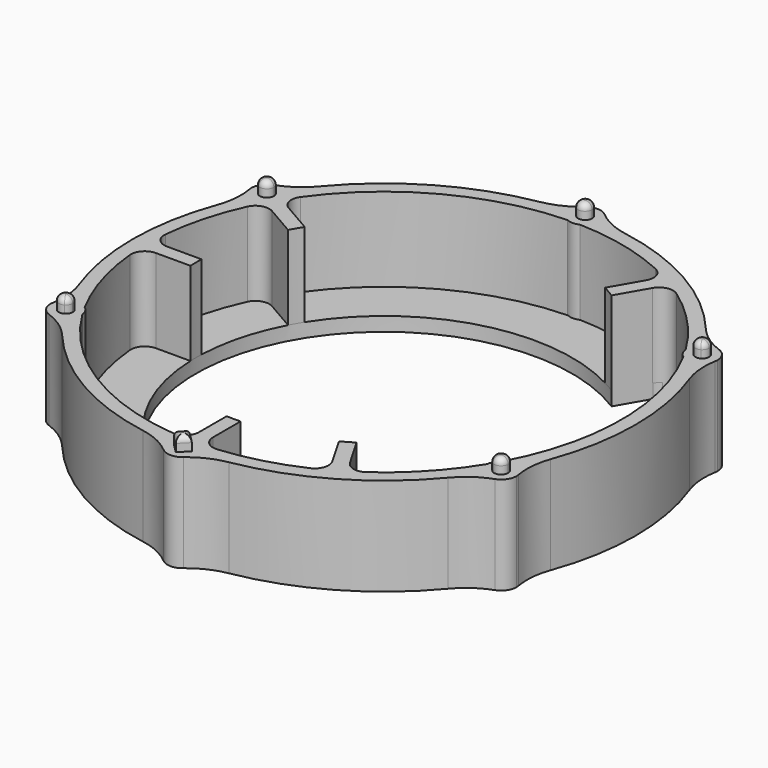
from build123d import *

# Parameters (mm, degrees)
F1_R          = 18
F1_R_2        = 17
F2_DEPTH      = 7
F3_DEPTH      = 7
F4_DEPTH      = 1
F6_DEPTH      = 7
F7_R          = 1
F8_R          = 5
F9_DEPTH      = 8
F10_R         = 0.44999
F11_DEPTH     = 1.8
F13_DEPTH     = 1
F12_R         = 13.47
F14_DEPTH     = 1
F15_T1_DEPTH  = 1
F15_T6_DEPTH  = 3.7422914514
F15_S7_R      = 1
F15_T8_DEPTH  = 4
F15_T12_DEPTH = 3.7422914514
F15_S13_R     = 1
F15_T14_DEPTH = 4
F15_T18_DEPTH = 3.7422914514
F15_S19_R     = 1
F15_T20_DEPTH = 4


# Not quite as in the source:
# - a fillet or chamfer that OpenCascade refuses, or shapes differently, is made with other operations: its cross-section is extruded or revolved along the edge and cut away or added
# - a fillet or chamfer is up to 0.001 mm smaller than in the source, because OpenCascade refuses the exact size


with BuildPart() as f2:
    # F1 (on Top) → F2 (new body)
    with BuildSketch(Plane.XY):
        Circle(F1_R)
        Circle(F1_R_2, mode=Mode.SUBTRACT)
    extrude(amount=F2_DEPTH)

    # F0 (on Top) → F3 (join)
    with BuildSketch(Plane.XY):
        with BuildLine():
            Line((-11.4073228059, 7.1633711619), (-14.4660626528, 8.9293354359))
            ThreePointArc((-14.4660626528, 8.9293354359), (-14.7224318643, 8.5), (-14.9660626528, 8.0633100321))
            Line((-14.9660626528, 8.0633100321), (-11.9073228059, 6.2973457581))
            ThreePointArc((-11.9073228059, 6.2973457581), (-11.665362189, 6.735), (-11.4073228059, 7.1633711619))
        make_face()
        with BuildLine():
            Line((7.1633711619, 11.4073228059), (8.9293354359, 14.4660626528))
            ThreePointArc((8.9293354359, 14.4660626528), (8.5, 14.7224318643), (8.0633100321, 14.9660626528))
            Line((8.0633100321, 14.9660626528), (6.2973457581, 11.9073228059))
            ThreePointArc((6.2973457581, 11.9073228059), (6.735, 11.665362189), (7.1633711619, 11.4073228059))
        make_face()
        with BuildLine():
            ThreePointArc((-0.5, -16.992645468), (0, -17), (0.5, -16.992645468))
            Line((0.5, -16.992645468), (0.5, -13.46071692))
            ThreePointArc((0.5, -13.46071692), (0, -13.47), (-0.5, -13.46071692))
            Line((-0.5, -13.46071692), (-0.5, -16.992645468))
        make_face()
        with BuildLine():
            ThreePointArc((8.0633100321, -14.9660626528), (8.5, -14.7224318643), (8.9293354359, -14.4660626528))
            Line((8.9293354359, -14.4660626528), (7.1633711619, -11.4073228059))
            ThreePointArc((7.1633711619, -11.4073228059), (6.735, -11.665362189), (6.2973457581, -11.9073228059))
            Line((6.2973457581, -11.9073228059), (8.0633100321, -14.9660626528))
        make_face()
        with BuildLine():
            Line((-13.46071692, 0.5), (-16.992645468, 0.5))
            ThreePointArc((-16.992645468, 0.5), (-17, 0), (-16.992645468, -0.5))
            Line((-16.992645468, -0.5), (-13.46071692, -0.5))
            ThreePointArc((-13.46071692, -0.5), (-13.47, 0), (-13.46071692, 0.5))
        make_face()
    extrude(amount=F3_DEPTH)

    # F1 (on Top) → F4 (join)
    with BuildSketch(Plane.XY):
        Circle(F1_R)
        Circle(F1_R_2, mode=Mode.SUBTRACT)
        Circle(F1_R_2)
    extrude(amount=F4_DEPTH)

    # F5 (on Top) → F6 (join)
    with BuildSketch(Plane.XY):
        with BuildLine():
            ThreePointArc((-14.4884572681, 9), (-14.6275367743, 9.5353800561), (-15.0096060035, 9.935377578))
            ThreePointArc((-15.0096060035, 9.935377578), (-15.1731450826, 9.6837837802), (-15.3324673166, 9.4294987133))
            ThreePointArc((-15.3324673166, 9.4294987133), (-15.153718855, 9.2469868663), (-15.0884572681, 9))
            ThreePointArc((-15.0884572681, 9), (-15.3354561915, 8.5687338928), (-15.832419089, 8.5635568422))
            ThreePointArc((-15.832419089, 8.5635568422), (-15.9729752997, 8.2984372068), (-16.1090923805, 8.0310113108))
            ThreePointArc((-16.1090923805, 8.0310113108), (-15.0239657375, 8.0558870238), (-14.4884572681, 9))
        make_face()
        with BuildLine():
            ThreePointArc((-15.3324673166, 9.4294987133), (-15.1731450826, 9.6837837802), (-15.0096060035, 9.935377578))
            ThreePointArc((-15.0096060035, 9.935377578), (-16.5410852123, 9.55), (-16.1090923805, 8.0310113108))
            ThreePointArc((-16.1090923805, 8.0310113108), (-15.9729752997, 8.2984372068), (-15.832419089, 8.5635568422))
            ThreePointArc((-15.832419089, 8.5635568422), (-16.02146997, 9.25), (-15.3324673166, 9.4294987133))
        make_face()
        with BuildLine():
            ThreePointArc((-1.099486377, 17.9663888889), (0, 16.9), (1.099486377, 17.9663888889))
            ThreePointArc((1.099486377, 17.9663888889), (0.7998302171, 17.982220987), (0.4999517724, 17.9930555556))
            ThreePointArc((0.4999517724, 17.9930555556), (0, 17.5), (-0.4999517724, 17.9930555556))
            ThreePointArc((-0.4999517724, 17.9930555556), (-0.7998302171, 17.982220987), (-1.099486377, 17.9663888889))
        make_face()
        with BuildLine():
            ThreePointArc((0.4999517724, 17.9930555556), (0.7998302171, 17.982220987), (1.099486377, 17.9663888889))
            ThreePointArc((1.099486377, 17.9663888889), (1.0998715868, 17.9831924823), (1.1, 18))
            ThreePointArc((1.1, 18), (-0.0168075177, 19.0998715868), (-1.099486377, 17.9663888889))
            ThreePointArc((-1.099486377, 17.9663888889), (-0.7998302171, 17.982220987), (-0.4999517724, 17.9930555556))
            ThreePointArc((-0.4999517724, 17.9930555556), (-0.003472306, 18.4999879429), (0.5, 18))
            ThreePointArc((0.5, 18), (0.4999879429, 17.996527694), (0.4999517724, 17.9930555556))
        make_face()
        with BuildLine():
            ThreePointArc((15.832419089, 8.5635568422), (15.9729752997, 8.2984372068), (16.1090923805, 8.0310113108))
            ThreePointArc((16.1090923805, 8.0310113108), (16.5325702443, 8.4355084694), (16.6884572681, 9))
            ThreePointArc((16.6884572681, 9), (16.1238373242, 9.9609204939), (15.0096060035, 9.935377578))
            ThreePointArc((15.0096060035, 9.935377578), (15.1731450826, 9.6837837802), (15.3324673166, 9.4294987133))
            ThreePointArc((15.3324673166, 9.4294987133), (15.8354441344, 9.4347384132), (16.0884572681, 9))
            ThreePointArc((16.0884572681, 9), (16.0197233753, 8.7469989234), (15.832419089, 8.5635568422))
        make_face()
        with BuildLine():
            ThreePointArc((15.0096060035, 9.935377578), (14.635829324, 8.45), (16.1090923805, 8.0310113108))
            ThreePointArc((16.1090923805, 8.0310113108), (15.9729752997, 8.2984372068), (15.832419089, 8.5635568422))
            ThreePointArc((15.832419089, 8.5635568422), (15.1554445662, 8.75), (15.3324673166, 9.4294987133))
            ThreePointArc((15.3324673166, 9.4294987133), (15.1731450826, 9.6837837802), (15.0096060035, 9.935377578))
        make_face()
        with BuildLine():
            ThreePointArc((-15.3324673166, -9.4294987133), (-15.1731450826, -9.6837837802), (-15.0096060035, -9.935377578))
            ThreePointArc((-15.0096060035, -9.935377578), (-14.6275367743, -9.5353800561), (-14.4884572681, -9))
            ThreePointArc((-14.4884572681, -9), (-15.0239657375, -8.0558870238), (-16.1090923805, -8.0310113108))
            ThreePointArc((-16.1090923805, -8.0310113108), (-15.9729752997, -8.2984372068), (-15.832419089, -8.5635568422))
            ThreePointArc((-15.832419089, -8.5635568422), (-15.3354561915, -8.5687338928), (-15.0884572681, -9))
            ThreePointArc((-15.0884572681, -9), (-15.153718855, -9.2469868663), (-15.3324673166, -9.4294987133))
        make_face()
        with BuildLine():
            ThreePointArc((-16.1090923805, -8.0310113108), (-16.5410852123, -9.55), (-15.0096060035, -9.935377578))
            ThreePointArc((-15.0096060035, -9.935377578), (-15.1731450826, -9.6837837802), (-15.3324673166, -9.4294987133))
            ThreePointArc((-15.3324673166, -9.4294987133), (-16.02146997, -9.25), (-15.832419089, -8.5635568422))
            ThreePointArc((-15.832419089, -8.5635568422), (-15.9729752997, -8.2984372068), (-16.1090923805, -8.0310113108))
        make_face()
        with BuildLine():
            ThreePointArc((0.6255239257, -17.9891278226), (0.8625800837, -17.9793202207), (1.099486377, -17.9663888889))
            ThreePointArc((1.099486377, -17.9663888889), (0, -16.9), (-1.099486377, -17.9663888889))
            ThreePointArc((-1.099486377, -17.9663888889), (-0.8625800837, -17.9793202207), (-0.6255239257, -17.9891278226))
            Line((-0.6255239257, -17.9891278226), (0, -17.3636038969))
            Line((0, -17.3636038969), (0.6255239257, -17.9891278226))
        make_face()
        with BuildLine():
            ThreePointArc((1.1, -18), (1.0998715868, -17.9831924823), (1.099486377, -17.9663888889))
            ThreePointArc((1.099486377, -17.9663888889), (0.8625800837, -17.9793202207), (0.6255239257, -17.9891278226))
            Line((0.6255239257, -17.9891278226), (0.6363961031, -18))
            Line((0.6363961031, -18), (0, -18.6363961031))
            Line((0, -18.6363961031), (-0.6363961031, -18))
            Line((-0.6363961031, -18), (-0.6255239257, -17.9891278226))
            ThreePointArc((-0.6255239257, -17.9891278226), (-0.8625800837, -17.9793202207), (-1.099486377, -17.9663888889))
            ThreePointArc((-1.099486377, -17.9663888889), (-0.0168075177, -19.0998715868), (1.1, -18))
        make_face()
        with BuildLine():
            ThreePointArc((16.6884572681, -9), (16.5325702443, -8.4355084694), (16.1090923805, -8.0310113108))
            ThreePointArc((16.1090923805, -8.0310113108), (15.9729752997, -8.2984372068), (15.832419089, -8.5635568422))
            ThreePointArc((15.832419089, -8.5635568422), (16.0197233753, -8.7469989234), (16.0884572681, -9))
            ThreePointArc((16.0884572681, -9), (15.8354441344, -9.4347384132), (15.3324673166, -9.4294987133))
            ThreePointArc((15.3324673166, -9.4294987133), (15.1731450826, -9.6837837802), (15.0096060035, -9.935377578))
            ThreePointArc((15.0096060035, -9.935377578), (16.1238373242, -9.9609204939), (16.6884572681, -9))
        make_face()
        with BuildLine():
            ThreePointArc((15.832419089, -8.5635568422), (15.9729752997, -8.2984372068), (16.1090923805, -8.0310113108))
            ThreePointArc((16.1090923805, -8.0310113108), (14.635829324, -8.45), (15.0096060035, -9.935377578))
            ThreePointArc((15.0096060035, -9.935377578), (15.1731450826, -9.6837837802), (15.3324673166, -9.4294987133))
            ThreePointArc((15.3324673166, -9.4294987133), (15.1554445662, -8.75), (15.832419089, -8.5635568422))
        make_face()
        with BuildLine():
            ThreePointArc((-15.0884572681, 9), (-15.153718855, 9.2469868663), (-15.3324673166, 9.4294987133))
            ThreePointArc((-15.3324673166, 9.4294987133), (-15.5884572681, 9), (-15.832419089, 8.5635568422))
            ThreePointArc((-15.832419089, 8.5635568422), (-15.3354561915, 8.5687338928), (-15.0884572681, 9))
        make_face()
        with BuildLine():
            ThreePointArc((-15.832419089, 8.5635568422), (-15.5884572681, 9), (-15.3324673166, 9.4294987133))
            ThreePointArc((-15.3324673166, 9.4294987133), (-16.02146997, 9.25), (-15.832419089, 8.5635568422))
        make_face()
        with BuildLine():
            ThreePointArc((-0.4999517724, 17.9930555556), (0, 18), (0.4999517724, 17.9930555556))
            ThreePointArc((0.4999517724, 17.9930555556), (0.4999879429, 17.996527694), (0.5, 18))
            ThreePointArc((0.5, 18), (-0.003472306, 18.4999879429), (-0.4999517724, 17.9930555556))
        make_face()
        with BuildLine():
            ThreePointArc((-0.4999517724, 17.9930555556), (0, 17.5), (0.4999517724, 17.9930555556))
            ThreePointArc((0.4999517724, 17.9930555556), (0, 18), (-0.4999517724, 17.9930555556))
        make_face()
        with BuildLine():
            ThreePointArc((15.3324673166, 9.4294987133), (15.5884572681, 9), (15.832419089, 8.5635568422))
            ThreePointArc((15.832419089, 8.5635568422), (16.0197233753, 8.7469989234), (16.0884572681, 9))
            ThreePointArc((16.0884572681, 9), (15.8354441344, 9.4347384132), (15.3324673166, 9.4294987133))
        make_face()
        with BuildLine():
            ThreePointArc((15.3324673166, 9.4294987133), (15.1554445662, 8.75), (15.832419089, 8.5635568422))
            ThreePointArc((15.832419089, 8.5635568422), (15.5884572681, 9), (15.3324673166, 9.4294987133))
        make_face()
        with BuildLine():
            ThreePointArc((16.0884572681, -9), (16.0197233753, -8.7469989234), (15.832419089, -8.5635568422))
            ThreePointArc((15.832419089, -8.5635568422), (15.5884572681, -9), (15.3324673166, -9.4294987133))
            ThreePointArc((15.3324673166, -9.4294987133), (15.8354441344, -9.4347384132), (16.0884572681, -9))
        make_face()
        with BuildLine():
            ThreePointArc((15.3324673166, -9.4294987133), (15.5884572681, -9), (15.832419089, -8.5635568422))
            ThreePointArc((15.832419089, -8.5635568422), (15.1554445662, -8.75), (15.3324673166, -9.4294987133))
        make_face()
        with BuildLine():
            Line((0.6363961031, -18), (0.6255239257, -17.9891278226))
            ThreePointArc((0.6255239257, -17.9891278226), (0, -18), (-0.6255239257, -17.9891278226))
            Line((-0.6255239257, -17.9891278226), (-0.6363961031, -18))
            Line((-0.6363961031, -18), (0, -18.6363961031))
            Line((0, -18.6363961031), (0.6363961031, -18))
        make_face()
        with BuildLine():
            ThreePointArc((-15.832419089, -8.5635568422), (-16.02146997, -9.25), (-15.3324673166, -9.4294987133))
            ThreePointArc((-15.3324673166, -9.4294987133), (-15.5884572681, -9), (-15.832419089, -8.5635568422))
        make_face()
        with BuildLine():
            ThreePointArc((-15.832419089, -8.5635568422), (-15.5884572681, -9), (-15.3324673166, -9.4294987133))
            ThreePointArc((-15.3324673166, -9.4294987133), (-15.153718855, -9.2469868663), (-15.0884572681, -9))
            ThreePointArc((-15.0884572681, -9), (-15.3354561915, -8.5687338928), (-15.832419089, -8.5635568422))
        make_face()
        with BuildLine():
            ThreePointArc((-0.6255239257, -17.9891278226), (0, -18), (0.6255239257, -17.9891278226))
            Line((0.6255239257, -17.9891278226), (0, -17.3636038969))
            Line((0, -17.3636038969), (-0.6255239257, -17.9891278226))
        make_face()
    extrude(amount=F6_DEPTH)

    # F7
    f7_edges = [f2.edges().sort_by_distance(p)[0] for p in [
        (0.5, -16.992645, 4),
        (8.06331, 14.966063, 4),
        (-16.992645, 0.5, 4),
        (8.929335, -14.466063, 4),
        (-14.466063, 8.929335, 4),
        (-0.5, -16.992645, 4),
        (-16.992645, -0.5, 4),
        (-14.966063, 8.06331, 4),
        (8.06331, -14.966063, 4),
        (8.929335, 14.466063, 4),
    ]]
    fillet(f7_edges, radius=F7_R)

    # F8 (call 1 of 12: OpenCascade refuses the feature's edges together)
    f8_edges = [f2.edges().sort_by_distance(p)[0] for p in [
        (-16.109092, 8.031011, 3.5),
    ]]
    fillet(f8_edges, radius=F8_R)

    # F8#2 (call 2 of 12)
    f8_2_edges = [f2.edges().sort_by_distance(p)[0] for p in [
        (-15.009606, 9.935378, 3.5),
    ]]
    fillet(f8_2_edges, radius=F8_R)

    # F8#3 (call 3 of 12)
    f8_3_edges = [f2.edges().sort_by_distance(p)[0] for p in [
        (-1.099486, 17.966389, 3.5),
    ]]
    fillet(f8_3_edges, radius=F8_R)

    # F8#4 (call 4 of 12)
    f8_4_edges = [f2.edges().sort_by_distance(p)[0] for p in [
        (1.099486, 17.966389, 3.5),
    ]]
    fillet(f8_4_edges, radius=F8_R)

    # F8#5 (call 5 of 12)
    f8_5_edges = [f2.edges().sort_by_distance(p)[0] for p in [
        (-15.009606, -9.935378, 3.5),
    ]]
    fillet(f8_5_edges, radius=F8_R)

    # F8#6 (call 6 of 12)
    f8_6_edges = [f2.edges().sort_by_distance(p)[0] for p in [
        (-16.109092, -8.031011, 3.5),
    ]]
    fillet(f8_6_edges, radius=F8_R)

    # F8#7 (call 7 of 12)
    f8_7_edges = [f2.edges().sort_by_distance(p)[0] for p in [
        (1.099486, -17.966389, 3.5),
    ]]
    fillet(f8_7_edges, radius=F8_R)

    # F8#8 (call 8 of 12)
    f8_8_edges = [f2.edges().sort_by_distance(p)[0] for p in [
        (-1.099486, -17.966389, 3.5),
    ]]
    fillet(f8_8_edges, radius=F8_R)

    # F8#10 (call 9 of 12)
    f8_10_edges = [f2.edges().sort_by_distance(p)[0] for p in [
        (15.009606, -9.935378, 3.5),
    ]]
    fillet(f8_10_edges, radius=F8_R)

    # F8#11 (call 10 of 12)
    f8_11_edges = [f2.edges().sort_by_distance(p)[0] for p in [
        (16.109092, 8.031011, 3.5),
    ]]
    fillet(f8_11_edges, radius=F8_R)

    # F8#12 (call 11 of 12)
    f8_12_edges = [f2.edges().sort_by_distance(p)[0] for p in [
        (15.009606, 9.935378, 3.5),
    ]]
    fillet(f8_12_edges, radius=F8_R)

    # F8#9 (call 12 of 12)
    f8_9_edges = [f2.edges().sort_by_distance(p)[0] for p in [
        (16.109092, -8.031011, 3.5),
    ]]
    fillet(f8_9_edges, radius=F8_R)

    # F5 (on Top) → F9 (join)
    with BuildSketch(Plane.XY):
        with BuildLine():
            ThreePointArc((-15.832419089, 8.5635568422), (-15.5884572681, 9), (-15.3324673166, 9.4294987133))
            ThreePointArc((-15.3324673166, 9.4294987133), (-16.02146997, 9.25), (-15.832419089, 8.5635568422))
        make_face()
        with BuildLine():
            ThreePointArc((-15.0884572681, 9), (-15.153718855, 9.2469868663), (-15.3324673166, 9.4294987133))
            ThreePointArc((-15.3324673166, 9.4294987133), (-15.5884572681, 9), (-15.832419089, 8.5635568422))
            ThreePointArc((-15.832419089, 8.5635568422), (-15.3354561915, 8.5687338928), (-15.0884572681, 9))
        make_face()
        with BuildLine():
            ThreePointArc((-0.4999517724, 17.9930555556), (0, 18), (0.4999517724, 17.9930555556))
            ThreePointArc((0.4999517724, 17.9930555556), (0.4999879429, 17.996527694), (0.5, 18))
            ThreePointArc((0.5, 18), (-0.003472306, 18.4999879429), (-0.4999517724, 17.9930555556))
        make_face()
        with BuildLine():
            ThreePointArc((-0.4999517724, 17.9930555556), (0, 17.5), (0.4999517724, 17.9930555556))
            ThreePointArc((0.4999517724, 17.9930555556), (0, 18), (-0.4999517724, 17.9930555556))
        make_face()
        with BuildLine():
            ThreePointArc((15.3324673166, 9.4294987133), (15.1554445662, 8.75), (15.832419089, 8.5635568422))
            ThreePointArc((15.832419089, 8.5635568422), (15.5884572681, 9), (15.3324673166, 9.4294987133))
        make_face()
        with BuildLine():
            ThreePointArc((15.3324673166, 9.4294987133), (15.5884572681, 9), (15.832419089, 8.5635568422))
            ThreePointArc((15.832419089, 8.5635568422), (16.0197233753, 8.7469989234), (16.0884572681, 9))
            ThreePointArc((16.0884572681, 9), (15.8354441344, 9.4347384132), (15.3324673166, 9.4294987133))
        make_face()
        with BuildLine():
            ThreePointArc((15.3324673166, -9.4294987133), (15.5884572681, -9), (15.832419089, -8.5635568422))
            ThreePointArc((15.832419089, -8.5635568422), (15.1554445662, -8.75), (15.3324673166, -9.4294987133))
        make_face()
        with BuildLine():
            ThreePointArc((16.0884572681, -9), (16.0197233753, -8.7469989234), (15.832419089, -8.5635568422))
            ThreePointArc((15.832419089, -8.5635568422), (15.5884572681, -9), (15.3324673166, -9.4294987133))
            ThreePointArc((15.3324673166, -9.4294987133), (15.8354441344, -9.4347384132), (16.0884572681, -9))
        make_face()
        with BuildLine():
            Line((0.6363961031, -18), (0.6255239257, -17.9891278226))
            ThreePointArc((0.6255239257, -17.9891278226), (0, -18), (-0.6255239257, -17.9891278226))
            Line((-0.6255239257, -17.9891278226), (-0.6363961031, -18))
            Line((-0.6363961031, -18), (0, -18.6363961031))
            Line((0, -18.6363961031), (0.6363961031, -18))
        make_face()
        with BuildLine():
            ThreePointArc((-0.6255239257, -17.9891278226), (0, -18), (0.6255239257, -17.9891278226))
            Line((0.6255239257, -17.9891278226), (0, -17.3636038969))
            Line((0, -17.3636038969), (-0.6255239257, -17.9891278226))
        make_face()
        with BuildLine():
            ThreePointArc((-15.832419089, -8.5635568422), (-16.02146997, -9.25), (-15.3324673166, -9.4294987133))
            ThreePointArc((-15.3324673166, -9.4294987133), (-15.5884572681, -9), (-15.832419089, -8.5635568422))
        make_face()
        with BuildLine():
            ThreePointArc((-15.832419089, -8.5635568422), (-15.5884572681, -9), (-15.3324673166, -9.4294987133))
            ThreePointArc((-15.3324673166, -9.4294987133), (-15.153718855, -9.2469868663), (-15.0884572681, -9))
            ThreePointArc((-15.0884572681, -9), (-15.3354561915, -8.5687338928), (-15.832419089, -8.5635568422))
        make_face()
    extrude(amount=F9_DEPTH)

    # F10 (radius 0.45 in the source; OpenCascade refuses exactly that, so slightly less here)
    f10_edges = [f2.edges().sort_by_distance(p)[0] for p in [
        (-15.844447, -8.570501, 8),
        (-15.344495, 9.436443, 8),
        (0.499952, 18.006944, 8),
        (15.344495, 9.436443, 8),
        (15.844447, -8.570501, 8),
        (0.318198, -17.681802, 8),
        (-0.318198, -18.318198, 8),
        (0.318198, -18.318198, 8),
        (-0.318198, -17.681802, 8),
    ]]
    fillet(f10_edges, radius=F10_R)

    # F5 (on Top) → F11 (cut)
    with BuildSketch(Plane.XY):
        with BuildLine():
            ThreePointArc((-15.832419089, -8.5635568422), (-16.02146997, -9.25), (-15.3324673166, -9.4294987133))
            ThreePointArc((-15.3324673166, -9.4294987133), (-15.5884572681, -9), (-15.832419089, -8.5635568422))
        make_face()
        with BuildLine():
            ThreePointArc((-15.832419089, -8.5635568422), (-15.5884572681, -9), (-15.3324673166, -9.4294987133))
            ThreePointArc((-15.3324673166, -9.4294987133), (-15.153718855, -9.2469868663), (-15.0884572681, -9))
            ThreePointArc((-15.0884572681, -9), (-15.3354561915, -8.5687338928), (-15.832419089, -8.5635568422))
        make_face()
        with BuildLine():
            Line((0.6363961031, -18), (0.6255239257, -17.9891278226))
            ThreePointArc((0.6255239257, -17.9891278226), (0, -18), (-0.6255239257, -17.9891278226))
            Line((-0.6255239257, -17.9891278226), (-0.6363961031, -18))
            Line((-0.6363961031, -18), (0, -18.6363961031))
            Line((0, -18.6363961031), (0.6363961031, -18))
        make_face()
        with BuildLine():
            ThreePointArc((-0.6255239257, -17.9891278226), (0, -18), (0.6255239257, -17.9891278226))
            Line((0.6255239257, -17.9891278226), (0, -17.3636038969))
            Line((0, -17.3636038969), (-0.6255239257, -17.9891278226))
        make_face()
        with BuildLine():
            ThreePointArc((15.3324673166, -9.4294987133), (15.5884572681, -9), (15.832419089, -8.5635568422))
            ThreePointArc((15.832419089, -8.5635568422), (15.1554445662, -8.75), (15.3324673166, -9.4294987133))
        make_face()
        with BuildLine():
            ThreePointArc((16.0884572681, -9), (16.0197233753, -8.7469989234), (15.832419089, -8.5635568422))
            ThreePointArc((15.832419089, -8.5635568422), (15.5884572681, -9), (15.3324673166, -9.4294987133))
            ThreePointArc((15.3324673166, -9.4294987133), (15.8354441344, -9.4347384132), (16.0884572681, -9))
        make_face()
        with BuildLine():
            ThreePointArc((15.3324673166, 9.4294987133), (15.1554445662, 8.75), (15.832419089, 8.5635568422))
            ThreePointArc((15.832419089, 8.5635568422), (15.5884572681, 9), (15.3324673166, 9.4294987133))
        make_face()
        with BuildLine():
            ThreePointArc((15.3324673166, 9.4294987133), (15.5884572681, 9), (15.832419089, 8.5635568422))
            ThreePointArc((15.832419089, 8.5635568422), (16.0197233753, 8.7469989234), (16.0884572681, 9))
            ThreePointArc((16.0884572681, 9), (15.8354441344, 9.4347384132), (15.3324673166, 9.4294987133))
        make_face()
        with BuildLine():
            ThreePointArc((-0.4999517724, 17.9930555556), (0, 17.5), (0.4999517724, 17.9930555556))
            ThreePointArc((0.4999517724, 17.9930555556), (0, 18), (-0.4999517724, 17.9930555556))
        make_face()
        with BuildLine():
            ThreePointArc((-0.4999517724, 17.9930555556), (0, 18), (0.4999517724, 17.9930555556))
            ThreePointArc((0.4999517724, 17.9930555556), (0.4999879429, 17.996527694), (0.5, 18))
            ThreePointArc((0.5, 18), (-0.003472306, 18.4999879429), (-0.4999517724, 17.9930555556))
        make_face()
        with BuildLine():
            ThreePointArc((-15.832419089, 8.5635568422), (-15.5884572681, 9), (-15.3324673166, 9.4294987133))
            ThreePointArc((-15.3324673166, 9.4294987133), (-16.02146997, 9.25), (-15.832419089, 8.5635568422))
        make_face()
        with BuildLine():
            ThreePointArc((-15.0884572681, 9), (-15.153718855, 9.2469868663), (-15.3324673166, 9.4294987133))
            ThreePointArc((-15.3324673166, 9.4294987133), (-15.5884572681, 9), (-15.832419089, 8.5635568422))
            ThreePointArc((-15.832419089, 8.5635568422), (-15.3354561915, 8.5687338928), (-15.0884572681, 9))
        make_face()
    extrude(amount=F11_DEPTH, mode=Mode.SUBTRACT)

    # F0 (on Top) → F13 (cut)
    with BuildSketch(Plane.XY):
        with BuildLine():
            ThreePointArc((0.5, -16.992645468), (4.3999237667, -16.4207390469), (8.0633100321, -14.9660626528))
            Line((8.0633100321, -14.9660626528), (6.2973457581, -11.9073228059))
            ThreePointArc((6.2973457581, -11.9073228059), (3.4862925375, -13.0110208801), (0.5, -13.46071692))
            Line((0.5, -13.46071692), (0.5, -16.992645468))
        make_face()
        with BuildLine():
            Line((13.46071692, 0.5), (16.992645468, 0.5))
            ThreePointArc((16.992645468, 0.5), (16.4207390469, 4.3999237667), (14.9660626528, 8.0633100321))
            Line((14.9660626528, 8.0633100321), (11.9073228059, 6.2973457581))
            ThreePointArc((11.9073228059, 6.2973457581), (13.0110208801, 3.4862925375), (13.46071692, 0.5))
        make_face()
        with BuildLine():
            Line((11.4073228059, 7.1633711619), (14.4660626528, 8.9293354359))
            ThreePointArc((14.4660626528, 8.9293354359), (12.0208152802, 12.0208152802), (8.9293354359, 14.4660626528))
            Line((8.9293354359, 14.4660626528), (7.1633711619, 11.4073228059))
            ThreePointArc((7.1633711619, 11.4073228059), (9.5247283426, 9.5247283426), (11.4073228059, 7.1633711619))
        make_face()
    extrude(amount=F13_DEPTH, mode=Mode.SUBTRACT)

    # F12 (on Top) → F14 (cut)
    with BuildSketch(Plane.XY):
        Circle(F12_R)
    extrude(amount=F14_DEPTH, mode=Mode.SUBTRACT)

    # F15: fillet of radius 1 on 6 edges, made by hand

    # F15_s2 → F15_t1 (join)
    with BuildSketch(Plane.XY):
        with BuildLine():
            ThreePointArc((15.4552761967, 7.0815279314), (14.8492573621, 7.618390795), (14.0443057446, 7.5315953132))
            Line((14.0443057446, 7.5315953132), (13.9942398184, 7.6183120412))
            ThreePointArc((13.9942398184, 7.6183120412), (14.4552182724, 7.8839961955), (14.9159967265, 8.15002676))
            Line((14.9159967265, 8.15002676), (15.0542143926, 8.1108038068))
            ThreePointArc((15.0542143926, 8.1108038068), (15.3080505243, 7.6208987998), (15.5463073157, 7.1232379212))
            Line((15.5463073157, 7.1232379212), (15.4552761967, 7.0815279314))
        make_face()
        with BuildLine():
            ThreePointArc((13.8604211846, 9.8438978431), (14.0223486455, 9.0506387054), (13.5447057446, 8.3969278967))
            Line((13.5447057446, 8.3969278967), (13.5947716708, 8.3102111688))
            ThreePointArc((13.5947716708, 8.3102111688), (14.0553501249, 8.5765881434), (14.516128579, 8.8426187079))
            Line((14.516128579, 8.8426187079), (14.5512693381, 8.9819301946))
            ThreePointArc((14.5512693381, 8.9819301946), (14.2539172225, 9.4467112365), (13.9420586548, 9.9018781098))
            Line((13.9420586548, 9.9018781098), (13.8604211846, 9.8438978431))
        make_face()
        with BuildLine():
            ThreePointArc((16.9254257746, 1.5948550121), (16.6690295004, 0.8269087166), (15.9285232099, 0.4996))
            Line((15.9285232099, 0.4996), (15.9285232099, 0.3994681476))
            ThreePointArc((15.9285232099, 0.3994681476), (16.4605843389, 0.3998681476), (16.992645468, 0.3998681476))
            Line((16.992645468, 0.3998681476), (17.0927340014, 0.5029450545))
            ThreePointArc((17.0927340014, 0.5029450545), (17.0676100363, 1.0541333018), (17.025116031, 1.6042486609))
            Line((17.025116031, 1.6042486609), (16.9254257746, 1.5948550121))
        make_face()
    extrude(amount=F15_T1_DEPTH)


with BuildPart() as f15_tool4:
    # F15_s5 → F15_t6 (new body)
    with BuildSketch(Plane.XY):
        with BuildLine():
            ThreePointArc((9.8438978431, 13.8604211846), (9.0506387054, 14.0223486455), (8.3969278967, 13.5447057446))
            Line((8.3969278967, 13.5447057446), (8.3102111688, 13.5947716708))
            ThreePointArc((8.3102111688, 13.5947716708), (8.5765881434, 14.0553501249), (8.8426187079, 14.516128579))
            Line((8.8426187079, 14.516128579), (8.9819301946, 14.5512693381))
            ThreePointArc((8.9819301946, 14.5512693381), (9.4467112365, 14.2539172225), (9.9018781098, 13.9420586548))
            Line((9.9018781098, 13.9420586548), (9.8438978431, 13.8604211846))
        make_face()
    extrude(amount=F15_T6_DEPTH)

    # F15_s7 → F15_t8 (cut, symmetric)
    with BuildSketch(Plane.XY.offset(1.9)):
        with Locations((9.2638042667, 13.0453796613)):
            Circle(F15_S7_R)
    extrude(amount=F15_T8_DEPTH, both=True, mode=Mode.SUBTRACT)


with BuildPart() as f2_1:
    add(f2.part)

    # F15_t3: union F15_tool4
    add(f15_tool4.part)


with BuildPart() as f15_tool10:
    # F15_s11 → F15_t12 (new body)
    with BuildSketch(Plane.XY):
        with BuildLine():
            ThreePointArc((7.5315953132, -14.0443057446), (7.618390795, -14.8492573621), (7.0815279314, -15.4552761967))
            Line((7.0815279314, -15.4552761967), (7.1232379212, -15.5463073157))
            ThreePointArc((7.1232379212, -15.5463073157), (7.6208987998, -15.3080505243), (8.1108038068, -15.0542143926))
            Line((8.1108038068, -15.0542143926), (8.15002676, -14.9159967265))
            ThreePointArc((8.15002676, -14.9159967265), (7.8839961955, -14.4552182725), (7.6183120412, -13.9942398184))
            Line((7.6183120412, -13.9942398184), (7.5315953132, -14.0443057446))
        make_face()
    extrude(amount=F15_T12_DEPTH)

    # F15_s13 → F15_t14 (cut, symmetric)
    with BuildSketch(Plane.XY.offset(1.9)):
        with Locations((6.6657280554, -14.5453796613)):
            Circle(F15_S13_R)
    extrude(amount=F15_T14_DEPTH, both=True, mode=Mode.SUBTRACT)


with BuildPart() as f2_2:
    add(f2_1.part)

    # F15_t9: union F15_tool10
    add(f15_tool10.part)


with BuildPart() as f15_tool16:
    # F15_s17 → F15_t18 (new body)
    with BuildSketch(Plane.XY):
        with BuildLine():
            ThreePointArc((0.4996, -15.9285232099), (0.8269087166, -16.6690295004), (1.5948550121, -16.9254257746))
            Line((1.5948550121, -16.9254257746), (1.6042486609, -17.025116031))
            ThreePointArc((1.6042486609, -17.025116031), (1.0541333018, -17.0676100363), (0.5029450545, -17.0927340014))
            Line((0.5029450545, -17.0927340014), (0.3998681476, -16.992645468))
            ThreePointArc((0.3998681476, -16.992645468), (0.3998681476, -16.4605843389), (0.3994681476, -15.9285232099))
            Line((0.3994681476, -15.9285232099), (0.4996, -15.9285232099))
        make_face()
    extrude(amount=F15_T18_DEPTH)

    # F15_s19 → F15_t20 (cut, symmetric)
    with BuildSketch(Plane.XY.offset(1.9)):
        with Locations((1.5, -15.9295323221)):
            Circle(F15_S19_R)
    extrude(amount=F15_T20_DEPTH, both=True, mode=Mode.SUBTRACT)


with BuildPart() as f2_3:
    add(f2_2.part)

    # F15_t15: union F15_tool16
    add(f15_tool16.part)


solid = f2_3.part
